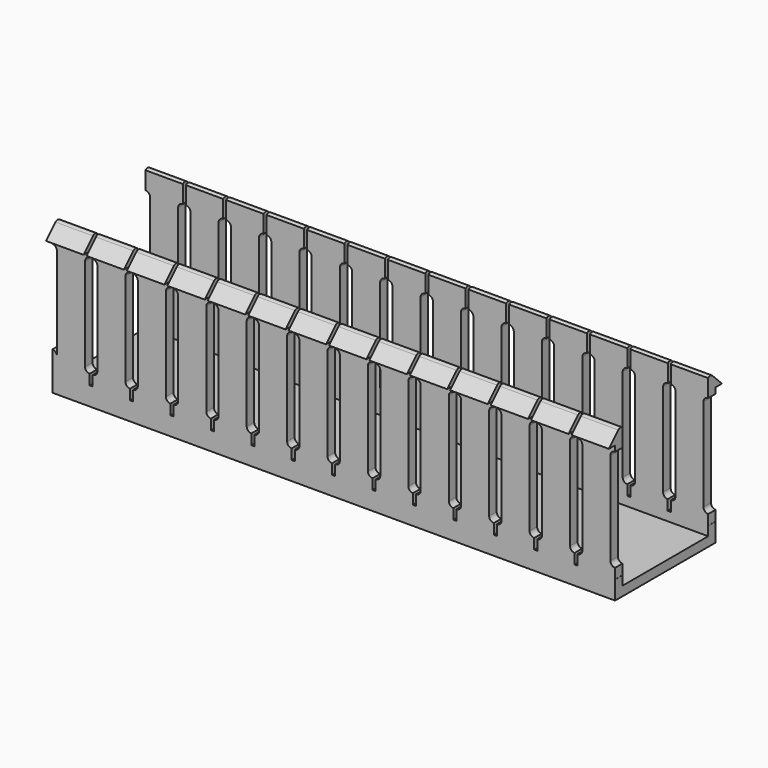
from build123d import *

# Parameters (mm, degrees)
F1_DEPTH      = 191.008
F2_W          = 1.016
F2_H          = 4.3925231637
F3_DEPTH      = 45.3146
F3_DEPTH_BACK = 2.6426


# Not quite as in the source:
# - ends of sketch curves that miss each other by under 0.0002 mm in the source are joined


with BuildPart() as f1:
    # F0 (on Right) → F1 (new body)
    with BuildSketch(Plane.YZ):
        with BuildLine():
            Line((0, 46.4074768363), (0, 0))
            Line((0, 0), (42.672, 0))
            Line((42.672, 0), (42.672, 46.4074768363))
            Line((42.672, 46.4074768363), (45.3136, 46.4074768363))
            Line((45.3136, 46.4074768363), (41.2930512242, 50.4280256121))
            ThreePointArc((41.2930512242, 50.4280256121), (40.3950256121, 50.8), (39.497, 50.4280256121))
            Line((39.497, 50.4280256121), (39.497, 3.175))
            Line((39.497, 3.175), (3.175, 3.175))
            Line((3.175, 3.175), (3.175, 50.4280256121))
            ThreePointArc((3.175, 50.4280256121), (2.2769743879, 50.8), (1.3789487758, 50.4280256121))
            Line((1.3789487758, 50.4280256121), (-2.6416, 46.4074768363))
            Line((-2.6416, 46.4074768363), (0, 46.4074768363))
        make_face()
    extrude(amount=F1_DEPTH)

    # F2 (on face) → F3 (cut, two sides)
    with BuildSketch(Plane.XZ) as f3_sk:
        with Locations((13.2080005054, 48.6037384182)):
            Rectangle(F2_W, F2_H)
        with BuildLine():
            Line((12.7000005054, 46.4074768363), (12.7000005054, 44.45))
            ThreePointArc((12.7000005054, 44.45), (11.5774681635, 43.9850321938), (11.1125, 42.8625))
            Line((11.1125, 42.8625), (11.1125, 11.3665))
            ThreePointArc((11.1125, 11.3665), (11.5661783059, 10.2552376515), (12.6679612754, 9.779))
            Line((12.6679612754, 9.779), (12.6679612754, 6.2915998527))
            Line((12.6679612754, 6.2915998527), (13.715999872, 6.2915998527))
            Line((13.715999872, 6.2915998527), (13.715999872, 9.779))
            ThreePointArc((13.715999872, 9.779), (14.8385318871, 10.2439679849), (15.303499872, 11.3665))
            Line((15.303499872, 11.3665), (15.303499872, 42.8625))
            ThreePointArc((15.303499872, 42.8625), (14.838532111, 43.9850317912), (13.7160005054, 44.45))
            Line((13.7160005054, 44.45), (13.7160005054, 46.4074768363))
            Line((13.7160005054, 46.4074768363), (12.7000005054, 46.4074768363))
        make_face()
        with Locations((26.9240003773, 48.6037384182)):
            Rectangle(F2_W, F2_H)
        with BuildLine():
            Line((27.4320003773, 46.4074768363), (26.4160003773, 46.4074768363))
            Line((26.4160003773, 46.4074768363), (26.4160003773, 44.45))
            ThreePointArc((26.4160003773, 44.45), (25.2934680355, 43.9850321938), (24.828499872, 42.8625))
            Line((24.828499872, 42.8625), (24.828499872, 11.3665))
            ThreePointArc((24.828499872, 11.3665), (25.2821781779, 10.2552376515), (26.3839611474, 9.779))
            Line((26.3839611474, 9.779), (26.3839611474, 6.2915998527))
            Line((26.3839611474, 6.2915998527), (27.431999744, 6.2915998527))
            Line((27.431999744, 6.2915998527), (27.431999744, 9.779))
            ThreePointArc((27.431999744, 9.779), (28.5545317591, 10.2439679849), (29.019499744, 11.3665))
            Line((29.019499744, 11.3665), (29.019499744, 42.8625))
            ThreePointArc((29.019499744, 42.8625), (28.554531983, 43.9850317912), (27.4320003773, 44.45))
            Line((27.4320003773, 44.45), (27.4320003773, 46.4074768363))
        make_face()
        with BuildLine():
            Line((1.5875, 11.3665), (1.5875, 42.8625))
            ThreePointArc((1.5875, 42.8625), (1.1225320151, 43.9850320151), (0, 44.45))
            Line((0, 44.45), (0, 42.8574001473))
            Line((0, 42.8574001473), (0, 12.9412487895))
            ThreePointArc((0, 12.9412487895), (1.1217525416, 12.4845328707), (1.5875, 11.3665))
        make_face()
        with BuildLine():
            Line((41.1480002493, 46.4074768363), (40.1320002493, 46.4074768363))
            Line((40.1320002493, 46.4074768363), (40.1320002493, 44.45))
            ThreePointArc((40.1320002493, 44.45), (39.0094679075, 43.9850321938), (38.544499744, 42.8625))
            Line((38.544499744, 42.8625), (38.544499744, 11.3665))
            ThreePointArc((38.544499744, 11.3665), (38.9981780499, 10.2552376515), (40.0999610193, 9.779))
            Line((40.0999610193, 9.779), (40.0999610193, 6.2915998527))
            Line((40.0999610193, 6.2915998527), (41.147999616, 6.2915998527))
            Line((41.147999616, 6.2915998527), (41.147999616, 9.779))
            ThreePointArc((41.147999616, 9.779), (42.2705316311, 10.2439679849), (42.735499616, 11.3665))
            Line((42.735499616, 11.3665), (42.735499616, 42.8625))
            ThreePointArc((42.735499616, 42.8625), (42.270531855, 43.9850317912), (41.1480002493, 44.45))
            Line((41.1480002493, 44.45), (41.1480002493, 46.4074768363))
        make_face()
        with Locations((40.6400002493, 48.6037384182)):
            Rectangle(F2_W, F2_H)
        with BuildLine():
            Line((54.8640001213, 46.4074768363), (53.8480001213, 46.4074768363))
            Line((53.8480001213, 46.4074768363), (53.8480001213, 44.45))
            ThreePointArc((53.8480001213, 44.45), (52.7254677795, 43.9850321938), (52.260499616, 42.8625))
            Line((52.260499616, 42.8625), (52.260499616, 11.3665))
            ThreePointArc((52.260499616, 11.3665), (52.7141779218, 10.2552376515), (53.8159608913, 9.779))
            Line((53.8159608913, 9.779), (53.8159608913, 6.2915998527))
            Line((53.8159608913, 6.2915998527), (54.8639994879, 6.2915998527))
            Line((54.8639994879, 6.2915998527), (54.8639994879, 9.779))
            ThreePointArc((54.8639994879, 9.779), (55.9865315031, 10.2439679849), (56.4514994879, 11.3665))
            Line((56.4514994879, 11.3665), (56.4514994879, 42.8625))
            ThreePointArc((56.4514994879, 42.8625), (55.986531727, 43.9850317912), (54.8640001213, 44.45))
            Line((54.8640001213, 44.45), (54.8640001213, 46.4074768363))
        make_face()
        with Locations((54.3560001213, 48.6037384182)):
            Rectangle(F2_W, F2_H)
        with BuildLine():
            Line((68.5799999933, 46.4074768363), (67.5639999933, 46.4074768363))
            Line((67.5639999933, 46.4074768363), (67.5639999933, 44.45))
            ThreePointArc((67.5639999933, 44.45), (66.4414676515, 43.9850321938), (65.9764994879, 42.8625))
            Line((65.9764994879, 42.8625), (65.9764994879, 11.3665))
            ThreePointArc((65.9764994879, 11.3665), (66.4301777938, 10.2552376515), (67.5319607633, 9.779))
            Line((67.5319607633, 9.779), (67.5319607633, 6.2915998527))
            Line((67.5319607633, 6.2915998527), (68.5799993599, 6.2915998527))
            Line((68.5799993599, 6.2915998527), (68.5799993599, 9.779))
            ThreePointArc((68.5799993599, 9.779), (69.7025313751, 10.2439679849), (70.1674993599, 11.3665))
            Line((70.1674993599, 11.3665), (70.1674993599, 42.8625))
            ThreePointArc((70.1674993599, 42.8625), (69.702531599, 43.9850317912), (68.5799999933, 44.45))
            Line((68.5799999933, 44.45), (68.5799999933, 46.4074768363))
        make_face()
        with Locations((68.0719999933, 48.6037384182)):
            Rectangle(F2_W, F2_H)
        with BuildLine():
            Line((82.2959998653, 46.4074768363), (81.2799998653, 46.4074768363))
            Line((81.2799998653, 46.4074768363), (81.2799998653, 44.45))
            ThreePointArc((81.2799998653, 44.45), (80.1574675235, 43.9850321938), (79.6924993599, 42.8625))
            Line((79.6924993599, 42.8625), (79.6924993599, 11.3665))
            ThreePointArc((79.6924993599, 11.3665), (80.1461776658, 10.2552376515), (81.2479606353, 9.779))
            Line((81.2479606353, 9.779), (81.2479606353, 6.2915998527))
            Line((81.2479606353, 6.2915998527), (82.2959992319, 6.2915998527))
            Line((82.2959992319, 6.2915998527), (82.2959992319, 9.779))
            ThreePointArc((82.2959992319, 9.779), (83.418531247, 10.2439679849), (83.8834992319, 11.3665))
            Line((83.8834992319, 11.3665), (83.8834992319, 42.8625))
            ThreePointArc((83.8834992319, 42.8625), (83.418531471, 43.9850317912), (82.2959998653, 44.45))
            Line((82.2959998653, 44.45), (82.2959998653, 46.4074768363))
        make_face()
        with Locations((81.7879998653, 48.6037384182)):
            Rectangle(F2_W, F2_H)
        with BuildLine():
            Line((96.0119997373, 46.4074768363), (94.9959997373, 46.4074768363))
            Line((94.9959997373, 46.4074768363), (94.9959997373, 44.45))
            ThreePointArc((94.9959997373, 44.45), (93.8734673955, 43.9850321938), (93.4084992319, 42.8625))
            Line((93.4084992319, 42.8625), (93.4084992319, 11.3665))
            ThreePointArc((93.4084992319, 11.3665), (93.8621775378, 10.2552376515), (94.9639605073, 9.779))
            Line((94.9639605073, 9.779), (94.9639605073, 6.2915998527))
            Line((94.9639605073, 6.2915998527), (96.0119991039, 6.2915998527))
            Line((96.0119991039, 6.2915998527), (96.0119991039, 9.779))
            ThreePointArc((96.0119991039, 9.779), (97.134531119, 10.2439679849), (97.5994991039, 11.3665))
            Line((97.5994991039, 11.3665), (97.5994991039, 42.8625))
            ThreePointArc((97.5994991039, 42.8625), (97.134531343, 43.9850317912), (96.0119997373, 44.45))
            Line((96.0119997373, 44.45), (96.0119997373, 46.4074768363))
        make_face()
        with Locations((95.5039997373, 48.6037384182)):
            Rectangle(F2_W, F2_H)
        with Locations((109.2199996093, 48.6037384182)):
            Rectangle(F2_W, F2_H)
        with Locations((122.9359994812, 48.6037384182)):
            Rectangle(F2_W, F2_H)
        with Locations((136.6519993532, 48.6037384182)):
            Rectangle(F2_W, F2_H)
        with Locations((150.3679992252, 48.6037384182)):
            Rectangle(F2_W, F2_H)
        with Locations((164.0839990972, 48.6037384182)):
            Rectangle(F2_W, F2_H)
        with Locations((177.7999989692, 48.6037384182)):
            Rectangle(F2_W, F2_H)
        with BuildLine():
            Line((190.9759596112, 6.2915998527), (191.008, 6.2915998527))
            Line((191.008, 6.2915998527), (191.008, 44.45))
            ThreePointArc((191.008, 44.45), (189.8854664994, 43.9850321938), (189.4204983358, 42.8625))
            Line((189.4204983358, 42.8625), (189.4204983358, 11.3665))
            ThreePointArc((189.4204983358, 11.3665), (189.8741766417, 10.2552376515), (190.9759596112, 9.779))
            Line((190.9759596112, 9.779), (190.9759596112, 6.2915998527))
        make_face()
        with BuildLine():
            Line((178.3079989692, 44.45), (178.3079989692, 46.4074768363))
            Line((178.3079989692, 46.4074768363), (177.2919989692, 46.4074768363))
            Line((177.2919989692, 46.4074768363), (177.2919989692, 44.45))
            ThreePointArc((177.2919989692, 44.45), (176.1694666274, 43.9850321938), (175.7044984638, 42.8625))
            Line((175.7044984638, 42.8625), (175.7044984638, 11.3665))
            ThreePointArc((175.7044984638, 11.3665), (176.1581767697, 10.2552376515), (177.2599597392, 9.779))
            Line((177.2599597392, 9.779), (177.2599597392, 6.2915998527))
            Line((177.2599597392, 6.2915998527), (178.3079983358, 6.2915998527))
            Line((178.3079983358, 6.2915998527), (178.3079983358, 9.779))
            ThreePointArc((178.3079983358, 9.779), (179.430530351, 10.2439679849), (179.8954983358, 11.3665))
            Line((179.8954983358, 11.3665), (179.8954983358, 42.8625))
            ThreePointArc((179.8954983358, 42.8625), (179.4305305749, 43.9850317912), (178.3079989692, 44.45))
        make_face()
        with BuildLine():
            Line((164.5919990972, 44.45), (164.5919990972, 46.4074768363))
            Line((164.5919990972, 46.4074768363), (163.5759990972, 46.4074768363))
            Line((163.5759990972, 46.4074768363), (163.5759990972, 44.45))
            ThreePointArc((163.5759990972, 44.45), (162.4534667554, 43.9850321938), (161.9884985918, 42.8625))
            Line((161.9884985918, 42.8625), (161.9884985918, 11.3665))
            ThreePointArc((161.9884985918, 11.3665), (162.4421768977, 10.2552376515), (163.5439598672, 9.779))
            Line((163.5439598672, 9.779), (163.5439598672, 6.2915998527))
            Line((163.5439598672, 6.2915998527), (164.5919984638, 6.2915998527))
            Line((164.5919984638, 6.2915998527), (164.5919984638, 9.779))
            ThreePointArc((164.5919984638, 9.779), (165.714530479, 10.2439679849), (166.1794984638, 11.3665))
            Line((166.1794984638, 11.3665), (166.1794984638, 42.8625))
            ThreePointArc((166.1794984638, 42.8625), (165.7145307029, 43.9850317912), (164.5919990972, 44.45))
        make_face()
        with BuildLine():
            Line((150.8759992252, 44.45), (150.8759992252, 46.4074768363))
            Line((150.8759992252, 46.4074768363), (149.8599992252, 46.4074768363))
            Line((149.8599992252, 46.4074768363), (149.8599992252, 44.45))
            ThreePointArc((149.8599992252, 44.45), (148.7374668834, 43.9850321938), (148.2724987199, 42.8625))
            Line((148.2724987199, 42.8625), (148.2724987199, 11.3665))
            ThreePointArc((148.2724987199, 11.3665), (148.7261770257, 10.2552376515), (149.8279599952, 9.779))
            Line((149.8279599952, 9.779), (149.8279599952, 6.2915998527))
            Line((149.8279599952, 6.2915998527), (150.8759985918, 6.2915998527))
            Line((150.8759985918, 6.2915998527), (150.8759985918, 9.779))
            ThreePointArc((150.8759985918, 9.779), (151.998530607, 10.2439679849), (152.4634985918, 11.3665))
            Line((152.4634985918, 11.3665), (152.4634985918, 42.8625))
            ThreePointArc((152.4634985918, 42.8625), (151.9985308309, 43.9850317912), (150.8759992252, 44.45))
        make_face()
        with BuildLine():
            Line((137.1599993532, 44.45), (137.1599993532, 46.4074768363))
            Line((137.1599993532, 46.4074768363), (136.1439993532, 46.4074768363))
            Line((136.1439993532, 46.4074768363), (136.1439993532, 44.45))
            ThreePointArc((136.1439993532, 44.45), (135.0214670114, 43.9850321938), (134.5564988479, 42.8625))
            Line((134.5564988479, 42.8625), (134.5564988479, 11.3665))
            ThreePointArc((134.5564988479, 11.3665), (135.0101771538, 10.2552376515), (136.1119601232, 9.779))
            Line((136.1119601232, 9.779), (136.1119601232, 6.2915998527))
            Line((136.1119601232, 6.2915998527), (137.1599987199, 6.2915998527))
            Line((137.1599987199, 6.2915998527), (137.1599987199, 9.779))
            ThreePointArc((137.1599987199, 9.779), (138.282530735, 10.2439679849), (138.7474987199, 11.3665))
            Line((138.7474987199, 11.3665), (138.7474987199, 42.8625))
            ThreePointArc((138.7474987199, 42.8625), (138.2825309589, 43.9850317912), (137.1599993532, 44.45))
        make_face()
        with BuildLine():
            Line((123.4439994812, 44.45), (123.4439994812, 46.4074768363))
            Line((123.4439994812, 46.4074768363), (122.4279994812, 46.4074768363))
            Line((122.4279994812, 46.4074768363), (122.4279994812, 44.45))
            ThreePointArc((122.4279994812, 44.45), (121.3054671394, 43.9850321938), (120.8404989759, 42.8625))
            Line((120.8404989759, 42.8625), (120.8404989759, 11.3665))
            ThreePointArc((120.8404989759, 11.3665), (121.2941772818, 10.2552376515), (122.3959602513, 9.779))
            Line((122.3959602513, 9.779), (122.3959602513, 6.2915998527))
            Line((122.3959602513, 6.2915998527), (123.4439988479, 6.2915998527))
            Line((123.4439988479, 6.2915998527), (123.4439988479, 9.779))
            ThreePointArc((123.4439988479, 9.779), (124.566530863, 10.2439679849), (125.0314988479, 11.3665))
            Line((125.0314988479, 11.3665), (125.0314988479, 42.8625))
            ThreePointArc((125.0314988479, 42.8625), (124.5665310869, 43.9850317912), (123.4439994812, 44.45))
        make_face()
        with BuildLine():
            Line((109.7279996093, 46.4074768363), (108.7119996093, 46.4074768363))
            Line((108.7119996093, 46.4074768363), (108.7119996093, 44.45))
            ThreePointArc((108.7119996093, 44.45), (107.5894672674, 43.9850321938), (107.1244991039, 42.8625))
            Line((107.1244991039, 42.8625), (107.1244991039, 11.3665))
            ThreePointArc((107.1244991039, 11.3665), (107.5781774098, 10.2552376515), (108.6799603793, 9.779))
            Line((108.6799603793, 9.779), (108.6799603793, 6.2915998527))
            Line((108.6799603793, 6.2915998527), (109.7279989759, 6.2915998527))
            Line((109.7279989759, 6.2915998527), (109.7279989759, 9.779))
            ThreePointArc((109.7279989759, 9.779), (110.850530991, 10.2439679849), (111.3154989759, 11.3665))
            Line((111.3154989759, 11.3665), (111.3154989759, 42.8625))
            ThreePointArc((111.3154989759, 42.8625), (110.850531215, 43.9850317912), (109.7279996093, 44.45))
            Line((109.7279996093, 44.45), (109.7279996093, 46.4074768363))
        make_face()
    extrude(amount=-F3_DEPTH, mode=Mode.SUBTRACT)
    extrude(f3_sk.sketch, amount=F3_DEPTH_BACK, mode=Mode.SUBTRACT)


solid = f1.part
